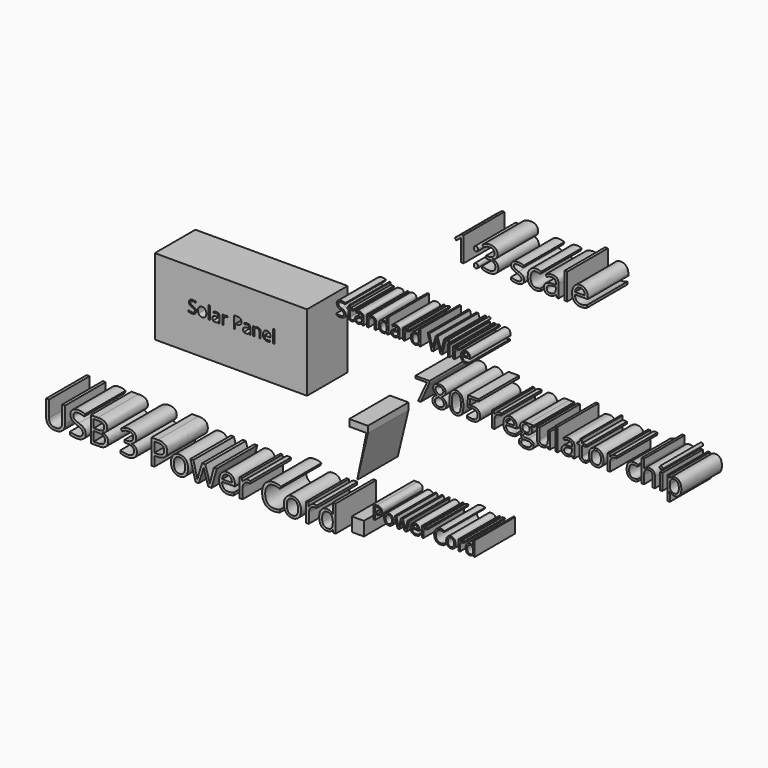
from build123d import *

# Parameters (mm, degrees)
F0_W           = 76.2
F0_H           = 38.1
F0_W_2         = 0.6837644207
F0_H_2         = 6.4068330983
F0_TEXT_SIZE   = 9.5947777502
F0_TEXT_SIZE_2 = 10.1762810344
F0_TEXT_SIZE_3 = 17.4417367412
F0_TEXT_SIZE_4 = 14.8508076866
F0_TEXT_SIZE_5 = 17.2946395146
F1_DEPTH       = 25.4


# Not quite as in the source:
# - Text() gives the source's letters only with a copy of the font that has no kerning and outlines rounded to 1/6400 em; it was checked with that copy


with BuildPart() as f1:
    # F0 (on Front) → F1 (new body)
    with BuildSketch(Plane.XZ):
        with Locations((-12.5604392118, 19.05)):
            Rectangle(F0_W, F0_H)
        with BuildLine():
            add(Edge.make_bspline(
                [(-25.4331834421, 21.5495263111), (-24.8752369447, 20.9191192296), (-24.8752369447, 19.84538512)],
                knots=[0, 0, 0, 1, 1, 1], degree=2))
            add(Edge.make_bspline(
                [(-24.8752369447, 19.84538512), (-24.8752369447, 18.7413493115), (-25.4305485118, 18.1214819513)],
                knots=[0, 0, 0, 1, 1, 1], degree=2))
            add(Edge.make_bspline(
                [(-25.4305485118, 18.1214819513), (-25.9858600789, 17.5016145911), (-26.9660541618, 17.5016145911)],
                knots=[0, 0, 0, 1, 1, 1], degree=2))
            add(Edge.make_bspline(
                [(-26.9660541618, 17.5016145911), (-27.5720881378, 17.5016145911), (-28.0411057366, 17.7861870668)],
                knots=[0, 0, 0, 1, 1, 1], degree=2))
            add(Edge.make_bspline(
                [(-28.0411057366, 17.7861870668), (-28.5101233354, 18.0707595425), (-28.7657115775, 18.601698004)],
                knots=[0, 0, 0, 1, 1, 1], degree=2))
            add(Edge.make_bspline(
                [(-28.7657115775, 18.601698004), (-29.0212998195, 19.1326364656), (-29.0212998195, 19.84538512)],
                knots=[0, 0, 0, 1, 1, 1], degree=2))
            add(Edge.make_bspline(
                [(-29.0212998195, 19.84538512), (-29.0212998195, 20.9481034632), (-28.4692819153, 21.5640184279)],
                knots=[0, 0, 0, 1, 1, 1], degree=2))
            add(Edge.make_bspline(
                [(-28.4692819153, 21.5640184279), (-27.9172640111, 22.1799333927), (-26.9370699282, 22.1799333927)],
                knots=[0, 0, 0, 1, 1, 1], degree=2))
            add(Edge.make_bspline(
                [(-26.9370699282, 22.1799333927), (-25.9911299396, 22.1799333927), (-25.4331834421, 21.5495263111)],
                knots=[0, 0, 0, 1, 1, 1], degree=2))
        make_face(mode=Mode.SUBTRACT)
        with BuildLine():
            Line((-18.2615618155, 17.5846148965), (-18.7687859041, 17.5846148965))
            Line((-18.7687859041, 17.5846148965), (-18.9044848161, 18.2275378971))
            Line((-18.9044848161, 18.2275378971), (-18.9374214452, 18.2275378971))
            add(Edge.make_bspline(
                [(-18.9374214452, 18.2275378971), (-19.2746925275, 17.8033141139), (-19.609987412, 17.6524643525)],
                knots=[0, 0, 0, 1, 1, 1], degree=2))
            add(Edge.make_bspline(
                [(-19.609987412, 17.6524643525), (-19.9452822966, 17.5016145911), (-20.4485539897, 17.5016145911)],
                knots=[0, 0, 0, 1, 1, 1], degree=2))
            add(Edge.make_bspline(
                [(-20.4485539897, 17.5016145911), (-21.1191437588, 17.5016145911), (-21.4998911915, 17.8481079296)],
                knots=[0, 0, 0, 1, 1, 1], degree=2))
            add(Edge.make_bspline(
                [(-21.4998911915, 17.8481079296), (-21.8806386242, 18.194601268), (-21.8806386242, 18.8322544079)],
                knots=[0, 0, 0, 1, 1, 1], degree=2))
            add(Edge.make_bspline(
                [(-21.8806386242, 18.8322544079), (-21.8806386242, 20.1984657842), (-19.6949639152, 20.2643390425)],
                knots=[0, 0, 0, 1, 1, 1], degree=2))
            Line((-19.6949639152, 20.2643390425), (-18.9295166542, 20.2893708806))
            Line((-18.9295166542, 20.2893708806), (-18.9295166542, 20.5699909608))
            add(Edge.make_bspline(
                [(-18.9295166542, 20.5699909608), (-18.9295166542, 21.1009294224), (-19.1574381278, 21.3538827341)],
                knots=[0, 0, 0, 1, 1, 1], degree=2))
            add(Edge.make_bspline(
                [(-19.1574381278, 21.3538827341), (-19.3853596014, 21.6068360458), (-19.8886312945, 21.6068360458)],
                knots=[0, 0, 0, 1, 1, 1], degree=2))
            add(Edge.make_bspline(
                [(-19.8886312945, 21.6068360458), (-20.4525063852, 21.6068360458), (-21.1639375744, 21.2616601725)],
                knots=[0, 0, 0, 1, 1, 1], degree=2))
            Line((-21.1639375744, 21.2616601725), (-21.3747320008, 21.7846938431))
            add(Edge.make_bspline(
                [(-21.3747320008, 21.7846938431), (-21.041413314, 21.9651865707), (-20.6441975667, 22.0679488536)],
                knots=[0, 0, 0, 1, 1, 1], degree=2))
            add(Edge.make_bspline(
                [(-20.6441975667, 22.0679488536), (-20.2469818194, 22.1707111365), (-19.8464724092, 22.1707111365)],
                knots=[0, 0, 0, 1, 1, 1], degree=2))
            add(Edge.make_bspline(
                [(-19.8464724092, 22.1707111365), (-19.0401837281, 22.1707111365), (-18.6508727718, 21.8130193442)],
                knots=[0, 0, 0, 1, 1, 1], degree=2))
            add(Edge.make_bspline(
                [(-18.6508727718, 21.8130193442), (-18.2615618155, 21.4553275518), (-18.2615618155, 20.6648484527)],
                knots=[0, 0, 0, 1, 1, 1], degree=2))
            Line((-18.2615618155, 20.6648484527), (-18.2615618155, 17.5846148965))
        make_face(mode=Mode.SUBTRACT)
        with BuildLine():
            add(Edge.make_bspline(
                [(-15.5739328785, 21.9408134652), (-15.2195347491, 22.1799333927), (-14.7953109659, 22.1799333927)],
                knots=[0, 0, 0, 1, 1, 1], degree=2))
            add(Edge.make_bspline(
                [(-14.7953109659, 22.1799333927), (-14.4949289082, 22.1799333927), (-14.2564677133, 22.1298697164)],
                knots=[0, 0, 0, 1, 1, 1], degree=2))
            Line((-14.2564677133, 22.1298697164), (-14.3513252052, 21.4961689719))
            add(Edge.make_bspline(
                [(-14.3513252052, 21.4961689719), (-14.6306278203, 21.5580898347), (-14.8453746422, 21.5580898347)],
                knots=[0, 0, 0, 1, 1, 1], degree=2))
            add(Edge.make_bspline(
                [(-14.8453746422, 21.5580898347), (-15.3934401509, 21.5580898347), (-15.7820923746, 21.1134453414)],
                knots=[0, 0, 0, 1, 1, 1], degree=2))
            add(Edge.make_bspline(
                [(-15.7820923746, 21.1134453414), (-16.1707445983, 20.6688008482), (-16.1707445983, 20.0061158701)],
                knots=[0, 0, 0, 1, 1, 1], degree=2))
            Line((-16.1707445983, 20.0061158701), (-16.1707445983, 17.5846148965))
            Line((-16.1707445983, 17.5846148965), (-16.8545090191, 17.5846148965))
            Line((-16.8545090191, 17.5846148965), (-16.8545090191, 22.0969330873))
            Line((-16.8545090191, 22.0969330873), (-16.2906339284, 22.0969330873))
            Line((-16.2906339284, 22.0969330873), (-16.2115860185, 21.2616601725))
            Line((-16.2115860185, 21.2616601725), (-16.1786493893, 21.2616601725))
            add(Edge.make_bspline(
                [(-16.1786493893, 21.2616601725), (-15.928331008, 21.7016935377), (-15.5739328785, 21.9408134652)],
                knots=[0, 0, 0, 1, 1, 1], degree=2))
        make_face(mode=Mode.SUBTRACT)
        with BuildLine():
            Line((-2.8630289649, 17.5846148965), (-3.3702530535, 17.5846148965))
            Line((-3.3702530535, 17.5846148965), (-3.5059519655, 18.2275378971))
            Line((-3.5059519655, 18.2275378971), (-3.5388885946, 18.2275378971))
            add(Edge.make_bspline(
                [(-3.5388885946, 18.2275378971), (-3.8761596769, 17.8033141139), (-4.2114545614, 17.6524643525)],
                knots=[0, 0, 0, 1, 1, 1], degree=2))
            add(Edge.make_bspline(
                [(-4.2114545614, 17.6524643525), (-4.546749446, 17.5016145911), (-5.0500211391, 17.5016145911)],
                knots=[0, 0, 0, 1, 1, 1], degree=2))
            add(Edge.make_bspline(
                [(-5.0500211391, 17.5016145911), (-5.7206109082, 17.5016145911), (-6.1013583409, 17.8481079296)],
                knots=[0, 0, 0, 1, 1, 1], degree=2))
            add(Edge.make_bspline(
                [(-6.1013583409, 17.8481079296), (-6.4821057736, 18.194601268), (-6.4821057736, 18.8322544079)],
                knots=[0, 0, 0, 1, 1, 1], degree=2))
            add(Edge.make_bspline(
                [(-6.4821057736, 18.8322544079), (-6.4821057736, 20.1984657842), (-4.2964310646, 20.2643390425)],
                knots=[0, 0, 0, 1, 1, 1], degree=2))
            Line((-4.2964310646, 20.2643390425), (-3.5309838036, 20.2893708806))
            Line((-3.5309838036, 20.2893708806), (-3.5309838036, 20.5699909608))
            add(Edge.make_bspline(
                [(-3.5309838036, 20.5699909608), (-3.5309838036, 21.1009294224), (-3.7589052772, 21.3538827341)],
                knots=[0, 0, 0, 1, 1, 1], degree=2))
            add(Edge.make_bspline(
                [(-3.7589052772, 21.3538827341), (-3.9868267508, 21.6068360458), (-4.4900984439, 21.6068360458)],
                knots=[0, 0, 0, 1, 1, 1], degree=2))
            add(Edge.make_bspline(
                [(-4.4900984439, 21.6068360458), (-5.0539735346, 21.6068360458), (-5.7654047238, 21.2616601725)],
                knots=[0, 0, 0, 1, 1, 1], degree=2))
            Line((-5.7654047238, 21.2616601725), (-5.9761991502, 21.7846938431))
            add(Edge.make_bspline(
                [(-5.9761991502, 21.7846938431), (-5.6428804634, 21.9651865707), (-5.2456647161, 22.0679488536)],
                knots=[0, 0, 0, 1, 1, 1], degree=2))
            add(Edge.make_bspline(
                [(-5.2456647161, 22.0679488536), (-4.8484489688, 22.1707111365), (-4.4479395586, 22.1707111365)],
                knots=[0, 0, 0, 1, 1, 1], degree=2))
            add(Edge.make_bspline(
                [(-4.4479395586, 22.1707111365), (-3.6416508775, 22.1707111365), (-3.2523399212, 21.8130193442)],
                knots=[0, 0, 0, 1, 1, 1], degree=2))
            add(Edge.make_bspline(
                [(-3.2523399212, 21.8130193442), (-2.8630289649, 21.4553275518), (-2.8630289649, 20.6648484527)],
                knots=[0, 0, 0, 1, 1, 1], degree=2))
            Line((-2.8630289649, 20.6648484527), (-2.8630289649, 17.5846148965))
        make_face(mode=Mode.SUBTRACT)
        with BuildLine():
            Line((2.3159265994, 17.5846148965), (1.6321621787, 17.5846148965))
            Line((1.6321621787, 17.5846148965), (1.6321621787, 20.5041177026))
            add(Edge.make_bspline(
                [(1.6321621787, 20.5041177026), (1.6321621787, 21.0548181416), (1.3811850647, 21.3268746982)],
                knots=[0, 0, 0, 1, 1, 1], degree=2))
            add(Edge.make_bspline(
                [(1.3811850647, 21.3268746982), (1.1302079508, 21.5989312548), (0.5939996285, 21.5989312548)],
                knots=[0, 0, 0, 1, 1, 1], degree=2))
            add(Edge.make_bspline(
                [(0.5939996285, 21.5989312548), (-0.1134791652, 21.5989312548), (-0.4428454564, 21.2162076243)],
                knots=[0, 0, 0, 1, 1, 1], degree=2))
            add(Edge.make_bspline(
                [(-0.4428454564, 21.2162076243), (-0.7722117477, 20.8334839938), (-0.7722117477, 19.9520997983)],
                knots=[0, 0, 0, 1, 1, 1], degree=2))
            Line((-0.7722117477, 19.9520997983), (-0.7722117477, 17.5846148965))
            Line((-0.7722117477, 17.5846148965), (-1.4559761685, 17.5846148965))
            Line((-1.4559761685, 17.5846148965), (-1.4559761685, 22.0969330873))
            Line((-1.4559761685, 22.0969330873), (-0.9000058688, 22.0969330873))
            Line((-0.9000058688, 22.0969330873), (-0.7893387949, 21.4790419248))
            Line((-0.7893387949, 21.4790419248), (-0.7564021658, 21.4790419248))
            add(Edge.make_bspline(
                [(-0.7564021658, 21.4790419248), (-0.5456077393, 21.8123606116), (-0.1668365043, 21.9961470021)],
                knots=[0, 0, 0, 1, 1, 1], degree=2))
            add(Edge.make_bspline(
                [(-0.1668365043, 21.9961470021), (0.2119347306, 22.1799333927), (0.676999934, 22.1799333927)],
                knots=[0, 0, 0, 1, 1, 1], degree=2))
            add(Edge.make_bspline(
                [(0.676999934, 22.1799333927), (1.4925108712, 22.1799333927), (1.9042187353, 21.7866700409)],
                knots=[0, 0, 0, 1, 1, 1], degree=2))
            add(Edge.make_bspline(
                [(1.9042187353, 21.7866700409), (2.3159265994, 21.393406689), (2.3159265994, 20.5278320755)],
                knots=[0, 0, 0, 1, 1, 1], degree=2))
            Line((2.3159265994, 20.5278320755), (2.3159265994, 17.5846148965))
        make_face(mode=Mode.SUBTRACT)
        with BuildLine():
            add(Edge.make_bspline(
                [(6.4053384722, 17.5701227797), (6.0825595067, 17.5016145911), (5.6253990944, 17.5016145911)],
                knots=[0, 0, 0, 1, 1, 1], degree=2))
            add(Edge.make_bspline(
                [(5.6253990944, 17.5016145911), (4.625443034, 17.5016145911), (4.0464170939, 18.1116009626)],
                knots=[0, 0, 0, 1, 1, 1], degree=2))
            add(Edge.make_bspline(
                [(4.0464170939, 18.1116009626), (3.4673911538, 18.7215873341), (3.4673911538, 19.8032262347)],
                knots=[0, 0, 0, 1, 1, 1], degree=2))
            add(Edge.make_bspline(
                [(3.4673911538, 19.8032262347), (3.4673911538, 20.8954048566), (4.0049169412, 21.5376691246)],
                knots=[0, 0, 0, 1, 1, 1], degree=2))
            add(Edge.make_bspline(
                [(4.0049169412, 21.5376691246), (4.5424427286, 22.1799333927), (5.4488587622, 22.1799333927)],
                knots=[0, 0, 0, 1, 1, 1], degree=2))
            add(Edge.make_bspline(
                [(5.4488587622, 22.1799333927), (6.2959888634, 22.1799333927), (6.7900383004, 21.6219868952)],
                knots=[0, 0, 0, 1, 1, 1], degree=2))
            add(Edge.make_bspline(
                [(6.7900383004, 21.6219868952), (7.2840877373, 21.0640403978), (7.2840877373, 20.1497195731)],
                knots=[0, 0, 0, 1, 1, 1], degree=2))
            Line((7.2840877373, 20.1497195731), (7.2840877373, 19.7175909989))
            Line((7.2840877373, 19.7175909989), (4.1761874127, 19.7175909989))
            add(Edge.make_bspline(
                [(4.1761874127, 19.7175909989), (4.1972668553, 18.9231595043), (4.578014288, 18.5114516402)],
                knots=[0, 0, 0, 1, 1, 1], degree=2))
            add(Edge.make_bspline(
                [(4.578014288, 18.5114516402), (4.9587617208, 18.0997437761), (5.6504309325, 18.0997437761)],
                knots=[0, 0, 0, 1, 1, 1], degree=2))
            add(Edge.make_bspline(
                [(5.6504309325, 18.0997437761), (6.3789891688, 18.0997437761), (7.090420358, 18.4040782293)],
                knots=[0, 0, 0, 1, 1, 1], degree=2))
            Line((7.090420358, 18.4040782293), (7.090420358, 17.7940918578))
            add(Edge.make_bspline(
                [(7.090420358, 17.7940918578), (6.7281174376, 17.6386309683), (6.4053384722, 17.5701227797)],
                knots=[0, 0, 0, 1, 1, 1], degree=2))
        make_face(mode=Mode.SUBTRACT)
        with BuildLine():
            add(Edge.make_bspline(
                [(-30.2544472141, 20.1905609932), (-29.8987316195, 19.8032262347), (-29.8987316195, 19.1866525374)],
                knots=[0, 0, 0, 1, 1, 1], degree=2))
            add(Edge.make_bspline(
                [(-29.8987316195, 19.1866525374), (-29.8987316195, 18.3922210428), (-30.4751226293, 17.9469178169)],
                knots=[0, 0, 0, 1, 1, 1], degree=2))
            add(Edge.make_bspline(
                [(-30.4751226293, 17.9469178169), (-31.051513639, 17.5016145911), (-32.0396125129, 17.5016145911)],
                knots=[0, 0, 0, 1, 1, 1], degree=2))
            add(Edge.make_bspline(
                [(-32.0396125129, 17.5016145911), (-33.109394227, 17.5016145911), (-33.6864439694, 17.7782822758)],
                knots=[0, 0, 0, 1, 1, 1], degree=2))
            Line((-33.6864439694, 17.7782822758), (-33.6864439694, 18.4528244404))
            add(Edge.make_bspline(
                [(-33.6864439694, 18.4528244404), (-33.3149187928, 18.2973635509), (-32.8788378231, 18.2064584545)],
                knots=[0, 0, 0, 1, 1, 1], degree=2))
            add(Edge.make_bspline(
                [(-32.8788378231, 18.2064584545), (-32.4427568535, 18.1155533581), (-32.0145806748, 18.1155533581)],
                knots=[0, 0, 0, 1, 1, 1], degree=2))
            add(Edge.make_bspline(
                [(-32.0145806748, 18.1155533581), (-31.3150066721, 18.1155533581), (-30.9606085426, 18.3810225889)],
                knots=[0, 0, 0, 1, 1, 1], degree=2))
            add(Edge.make_bspline(
                [(-30.9606085426, 18.3810225889), (-30.6062104132, 18.6464918197), (-30.6062104132, 19.1207792791)],
                knots=[0, 0, 0, 1, 1, 1], degree=2))
            add(Edge.make_bspline(
                [(-30.6062104132, 19.1207792791), (-30.6062104132, 19.4330185233), (-30.7320283365, 19.6326144958)],
                knots=[0, 0, 0, 1, 1, 1], degree=2))
            add(Edge.make_bspline(
                [(-30.7320283365, 19.6326144958), (-30.8578462598, 19.8322104683), (-31.1522997242, 20.001504742)],
                knots=[0, 0, 0, 1, 1, 1], degree=2))
            add(Edge.make_bspline(
                [(-31.1522997242, 20.001504742), (-31.4467531886, 20.1707990158), (-32.0475173039, 20.3842283725)],
                knots=[0, 0, 0, 1, 1, 1], degree=2))
            add(Edge.make_bspline(
                [(-32.0475173039, 20.3842283725), (-32.8867426141, 20.6846104302), (-33.2470693368, 21.0963182943)],
                knots=[0, 0, 0, 1, 1, 1], degree=2))
            add(Edge.make_bspline(
                [(-33.2470693368, 21.0963182943), (-33.6073960595, 21.5080261584), (-33.6073960595, 22.1707111365)],
                knots=[0, 0, 0, 1, 1, 1], degree=2))
            add(Edge.make_bspline(
                [(-33.6073960595, 22.1707111365), (-33.6073960595, 22.8663327437), (-33.0850211215, 23.2780406078)],
                knots=[0, 0, 0, 1, 1, 1], degree=2))
            add(Edge.make_bspline(
                [(-33.0850211215, 23.2780406078), (-32.5626461835, 23.689748472), (-31.7010239655, 23.689748472)],
                knots=[0, 0, 0, 1, 1, 1], degree=2))
            add(Edge.make_bspline(
                [(-31.7010239655, 23.689748472), (-30.803830188, 23.689748472), (-30.0502401135, 23.3603821807)],
                knots=[0, 0, 0, 1, 1, 1], degree=2))
            Line((-30.0502401135, 23.3603821807), (-30.2689393309, 22.7517132743))
            add(Edge.make_bspline(
                [(-30.2689393309, 22.7517132743), (-31.0146246144, 23.0639525185), (-31.7181510126, 23.0639525185)],
                knots=[0, 0, 0, 1, 1, 1], degree=2))
            add(Edge.make_bspline(
                [(-31.7181510126, 23.0639525185), (-32.2741213123, 23.0639525185), (-32.5870192891, 22.8254913236)],
                knots=[0, 0, 0, 1, 1, 1], degree=2))
            add(Edge.make_bspline(
                [(-32.5870192891, 22.8254913236), (-32.8999172658, 22.5870301287), (-32.8999172658, 22.1628063455)],
                knots=[0, 0, 0, 1, 1, 1], degree=2))
            add(Edge.make_bspline(
                [(-32.8999172658, 22.1628063455), (-32.8999172658, 21.8505671014), (-32.7846390638, 21.6503123963)],
                knots=[0, 0, 0, 1, 1, 1], degree=2))
            add(Edge.make_bspline(
                [(-32.7846390638, 21.6503123963), (-32.6693608619, 21.4500576912), (-32.3953281075, 21.2833983478)],
                knots=[0, 0, 0, 1, 1, 1], degree=2))
            add(Edge.make_bspline(
                [(-32.3953281075, 21.2833983478), (-32.1212953532, 21.1167390044), (-31.5574202625, 20.9151668341)],
                knots=[0, 0, 0, 1, 1, 1], degree=2))
            add(Edge.make_bspline(
                [(-31.5574202625, 20.9151668341), (-30.6101628087, 20.5778957518), (-30.2544472141, 20.1905609932)],
                knots=[0, 0, 0, 1, 1, 1], degree=2))
        make_face(mode=Mode.SUBTRACT)
        with Locations((-23.334461434, 20.7880314456)):
            Rectangle(F0_W_2, F0_H_2, mode=Mode.SUBTRACT)
        with BuildLine():
            add(Edge.make_bspline(
                [(-9.5570694692, 23.6041132362), (-7.3015691064, 23.6041132362), (-7.3015691064, 21.8505671014)],
                knots=[0, 0, 0, 1, 1, 1], degree=2))
            add(Edge.make_bspline(
                [(-7.3015691064, 21.8505671014), (-7.3015691064, 20.9362462767), (-7.9253888621, 20.4441730375)],
                knots=[0, 0, 0, 1, 1, 1], degree=2))
            add(Edge.make_bspline(
                [(-7.9253888621, 20.4441730375), (-8.5492086178, 19.9520997983), (-9.7098954283, 19.9520997983)],
                knots=[0, 0, 0, 1, 1, 1], degree=2))
            Line((-9.7098954283, 19.9520997983), (-10.4186916872, 19.9520997983))
            Line((-10.4186916872, 19.9520997983), (-10.4186916872, 17.5846148965))
            Line((-10.4186916872, 17.5846148965), (-11.1182656899, 17.5846148965))
            Line((-11.1182656899, 17.5846148965), (-11.1182656899, 23.6041132362))
            Line((-11.1182656899, 23.6041132362), (-9.5570694692, 23.6041132362))
        make_face(mode=Mode.SUBTRACT)
        with Locations((8.7919266189, 20.7880314456)):
            Rectangle(F0_W_2, F0_H_2, mode=Mode.SUBTRACT)
        Polygon((54.0098896683, -45.8456025943), (50.6604349816, -45.8456025943), (47.939005957, -45.8456025943), (47.939005957, -52.7538425745), (54.0098896683, -52.7538425745), align=None)
        Polygon((55.9961270933, -3.312318913), (46.6829630933, -3.312318913), (46.6829630933, -6.698900913), (55.2896339069, -6.698900913), align=None)
        Polygon((55.9961270933, -4.9775806256), (55.9961270933, -3.312318913), (55.2896339069, -6.698900913), (55.9961270933, -6.698900913), align=None)
        Polygon((55.9961270933, -6.698900913), (55.2896339069, -6.698900913), (50.6604349816, -28.8890112447), align=None)
        with Locations((57.7780224894, -43.7521950014)):
            Text('Power Cord', F0_TEXT_SIZE, font='Open Sans', text_align=(TextAlign.LEFT, TextAlign.BOTTOM))
        with Locations((39.7747273433, 40.1468099529)):
            Text('Standard Wire', F0_TEXT_SIZE_2, font='Open Sans', text_align=(TextAlign.LEFT, TextAlign.BOTTOM))
        with Locations((-106.663714163, -56.1308562756)):
            Text('USB 3 Power Cord', F0_TEXT_SIZE_3, font='Open Sans', text_align=(TextAlign.LEFT, TextAlign.BOTTOM))
        with Locations((79.0600180626, 15.8545169979)):
            Text('7805 regulator chip', F0_TEXT_SIZE_4, font='Open Sans', text_align=(TextAlign.LEFT, TextAlign.BOTTOM))
        with Locations((97.9051142931, 83.872616291)):
            Text('1:3 scale', F0_TEXT_SIZE_5, font='Open Sans', text_align=(TextAlign.LEFT, TextAlign.BOTTOM))
    extrude(amount=F1_DEPTH)


solid = f1.part
